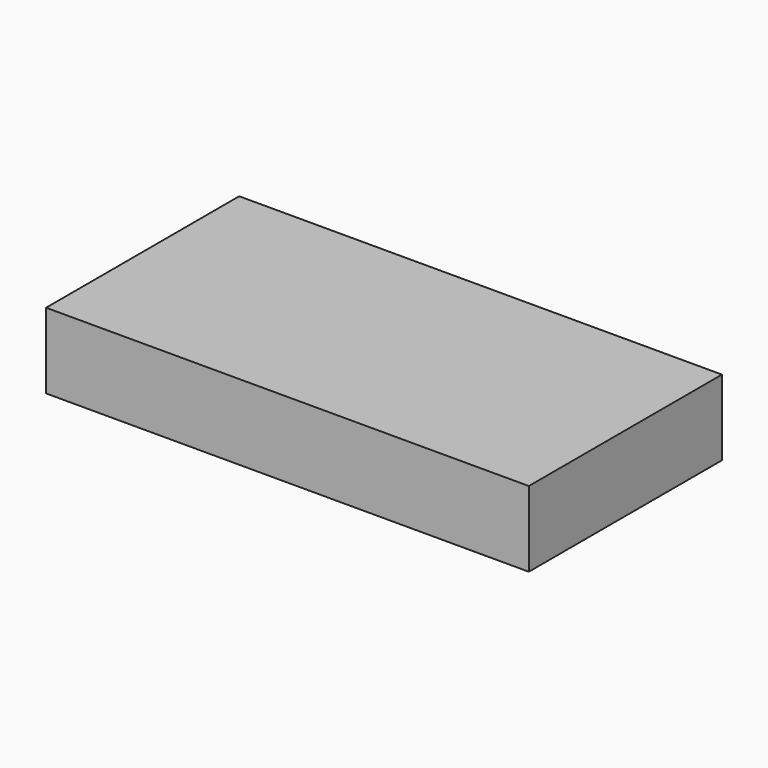
from build123d import *

# Parameters (mm, degrees)
F0_W     = 32.004
F0_H     = 16.002
F1_DEPTH = 5.0038


# Not quite as in the source:
# - the program builds the solid bodies; features that only make, move or delete a surface that nothing else refers to are left out


with BuildPart() as f1:
    # F0 (on Top) → F1 (new body)
    with BuildSketch(Plane.XY):
        with Locations((16.002, 8.001)):
            Rectangle(F0_W, F0_H)
    extrude(amount=F1_DEPTH)


solid = f1.part
